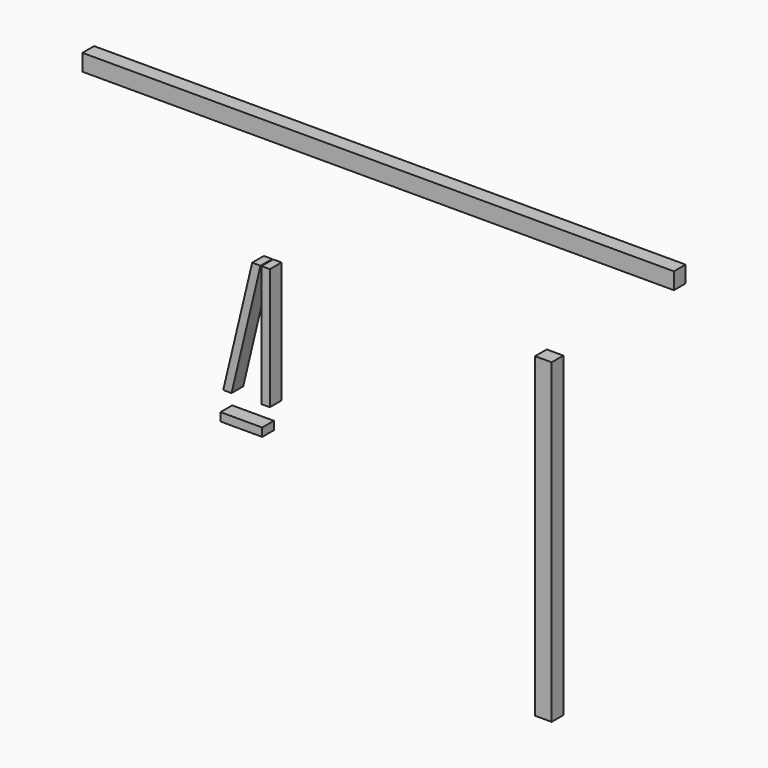
from build123d import *

# Parameters (mm, degrees)
F1_DEPTH = 44.45
F0_W     = 127
F0_H     = 25.4
F0_W_2   = 50.8
F0_H_2   = 965.2
F0_W_3   = 1803.4
F0_H_3   = 50.8
F0_W_4   = 25.4
F0_H_4   = 370.6241


# Not quite as in the source:
# - a feature names something its author has since deleted; it is built from what else it names


with BuildPart() as f1:
    # F0 (on Front) → F1 (new body)
    with BuildSketch(Plane.XZ):
        Polygon((316.756593769, 370.624931355), (228.4494012073, 0), (253.8494012073, 0), (342.156593769, 370.624931355), align=None)
    extrude(amount=F1_DEPTH)


with BuildPart() as f1b:
    # F0 (on Front) → F1, piece 2 (new body)
    with BuildSketch(Plane.XZ):
        with Locations((283.7561050653, -74.5373453617)):
            Rectangle(F0_W, F0_H)
    extrude(amount=F1_DEPTH)


with BuildPart() as f1c:
    # F0 (on Front) → F1, piece 3 (new body)
    with BuildSketch(Plane.XZ):
        with Locations((1204.4791366577, -82.4821556568)):
            Rectangle(F0_W_2, F0_H_2)
    extrude(amount=F1_DEPTH)


with BuildPart() as f1d:
    # F0 (on Front) → F1, piece 4 (new body)
    with BuildSketch(Plane.XZ):
        with Locations((700.8411536932, 740.1225183487)):
            Rectangle(F0_W_3, F0_H_3)
    extrude(amount=F1_DEPTH)


with BuildPart() as f1e:
    # F0 (on Front) → F1, piece 5 (new body)
    with BuildSketch(Plane.XZ):
        with Locations((357.8362252235, 185.31205)):
            Rectangle(F0_W_4, F0_H_4)
    extrude(amount=F1_DEPTH)


solid = Compound([f1.part, f1b.part, f1c.part, f1d.part, f1e.part])
